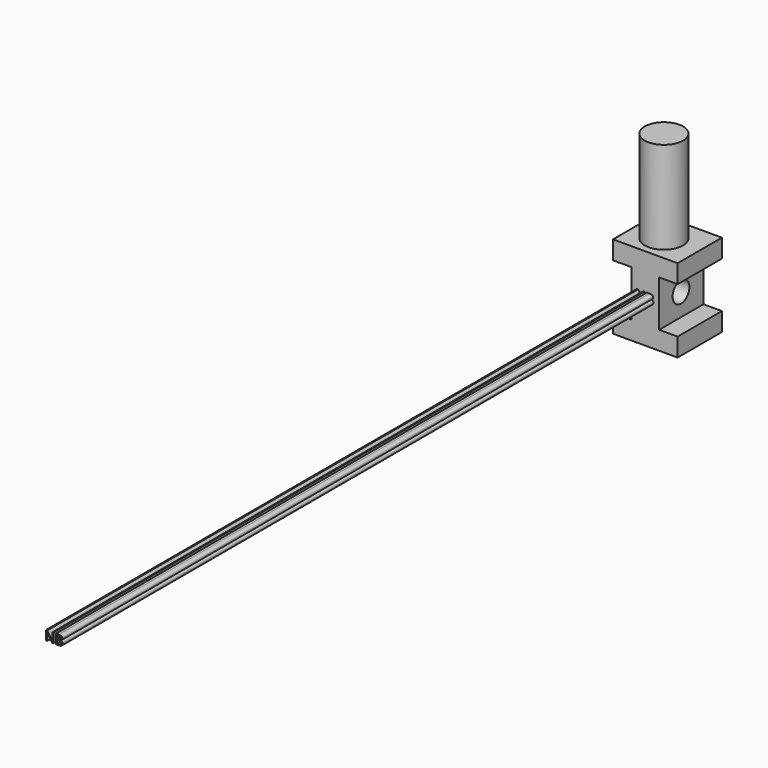
from build123d import *

# Parameters (mm, degrees)
F1_DEPTH     = 76.2
F2_R         = 14.410883718
F3_DEPTH     = 25.4
F4_DEPTH     = 25.4
F5_R         = 26.4071195409
F6_DEPTH     = 127
F7_TEXT_SIZE = 18.2134435616
F8_DEPTH     = 1016


# Not quite as in the source:
# - Text() gives the source's letters only with a copy of the font that has no kerning and outlines rounded to 1/6400 em; it was checked with that copy


with BuildPart() as f1:
    # F0 (on Front) → F1 (new body)
    with BuildSketch(Plane.XZ):
        Polygon((-41.3259547919, -26.6034284378), (-41.3259547919, -52.0034284378), (47.5740452081, -52.0034284378), (47.5740452081, -26.6034284378), (22.1740452081, -26.6034284378), (22.1740452081, 36.8965715622), (47.5740452081, 36.8965715622), (47.5740452081, 62.2965715622), (-41.3259547919, 62.2965715622), (-41.3259547919, 36.8965715622), (-15.9259547919, 36.8965715622), (-15.9259547919, -26.6034284378), align=None)
    extrude(amount=F1_DEPTH)

    # F2 (on face) → F3 (cut)
    with BuildSketch(Plane(origin=(-15.9259547919, 0, 0), x_dir=(0, -1, 0), z_dir=(-1, 0, 0))):
        with Locations((38.5907158566, 4.1584046951)):
            Circle(F2_R)
    extrude(amount=-F3_DEPTH, mode=Mode.SUBTRACT)

    # F4 (cut): a face of the model
    f4_faces = [f1.faces().sort_by_distance(p)[0] for p in [
        (9.4740452081, -38.5907158566, 4.1584046951),
    ]]
    extrude(f4_faces, amount=-F4_DEPTH, mode=Mode.SUBTRACT)

    # F5 (on face) → F6 (join)
    with BuildSketch(Plane.XY.offset(62.2965715622)):
        with Locations((0, -40.2406789362)):
            Circle(F5_R)
    extrude(amount=F6_DEPTH)

    # F7 (on face) → F8 (join)
    with BuildSketch(Plane.XZ.offset(76.2)):
        with Locations((-10.2349273762, 0)):
            Text('NB', F7_TEXT_SIZE, font='Open Sans', text_align=(TextAlign.LEFT, TextAlign.BOTTOM))
    extrude(amount=F8_DEPTH)


solid = f1.part
